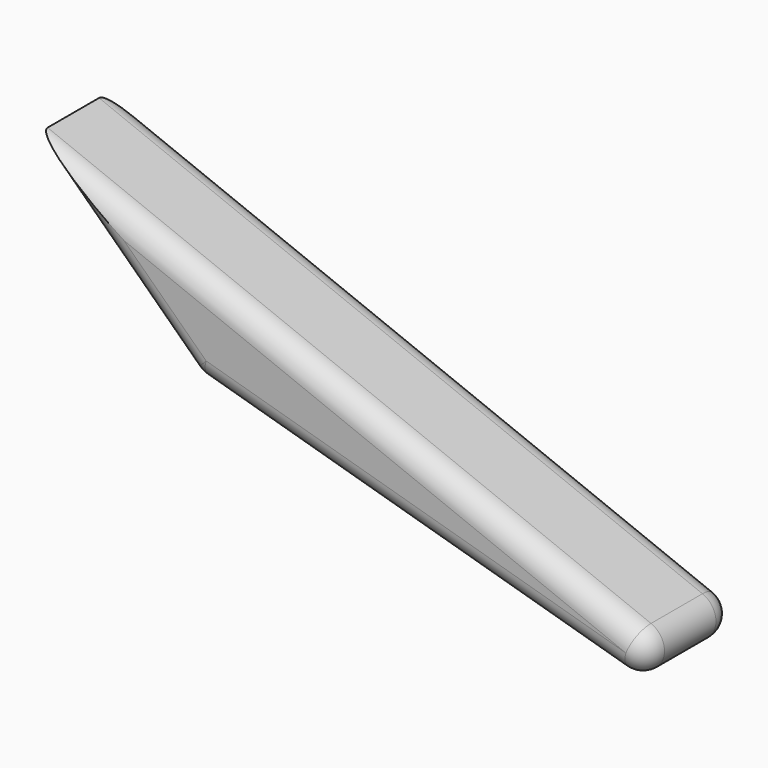
from build123d import *

# Parameters (mm, degrees)
F1_DEPTH = 25.4
F3_R     = 5.08


# Not quite as in the source:
# - a feature of the source that left no trace in its solid (it failed there, or was rolled back) is left out


with BuildPart() as f1:
    # F0 (on Front) → F1 (new body)
    with BuildSketch(Plane.XZ):
        Polygon((199.189722538, -57.2593323886), (-38.9998517931, 37.592638284), (0, 0), align=None)
    extrude(amount=F1_DEPTH)

    # F3
    f3_edges = [f1.edges().sort_by_distance(p)[0] for p in [
        (80.094935, -25.4, -9.833347),
        (-19.499926, -25.4, 18.796319),
        (99.594861, -25.4, -28.629666),
        (0, -12.7, 0),
        (199.189723, -12.7, -57.259332),
        (99.594861, 0, -28.629666),
        (80.094935, 0, -9.833347),
        (-19.499926, 0, 18.796319),
    ]]
    fillet(f3_edges, radius=F3_R)


solid = f1.part
